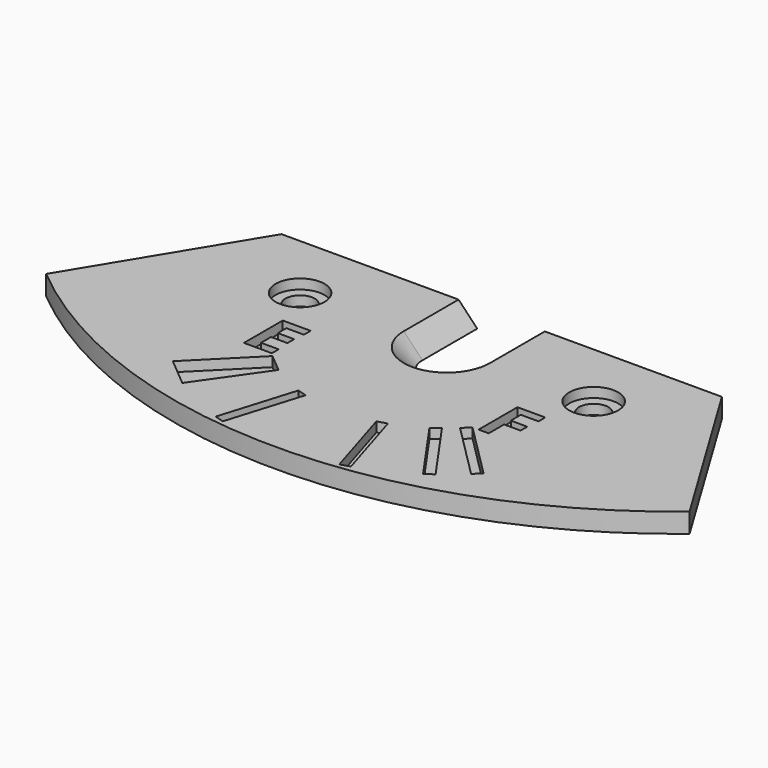
from build123d import *

# Parameters (mm, degrees)
F0_R         = 1.5
F1_DEPTH     = 2
F2_R         = 2.5
F2_R_2       = 1.5
F2_TEXT_SIZE = 6.9444444444
F3_DEPTH     = 1


# Not quite as in the source:
# - Text() gives the source's letters only with a copy of the font that has no kerning and outlines rounded to 1/6400 em; it was checked with that copy


with BuildPart() as f1:
    # F0 (on Top) → F1 (new body)
    with BuildSketch(Plane.XY):
        with BuildLine():
            ThreePointArc((2.5, 0), (0, -2.5), (-2.5, 0))
            Line((-2.5, 0), (-2.5, 7))
            Line((-2.5, 7), (-22.5, 7))
            Line((-22.5, 7), (-32.8723314143, -10.1001386261))
            ThreePointArc((-32.8723314143, -10.1001386261), (0, -22), (32.8723314143, -10.1001386261))
            Line((32.8723314143, -10.1001386261), (22.5, 7))
            Line((22.5, 7), (2.5, 7))
            Line((2.5, 7), (2.5, 0))
        make_face()
        with Locations((-15, 0)):
            Circle(F0_R, mode=Mode.SUBTRACT)
        with Locations((15, 0)):
            Circle(F0_R, mode=Mode.SUBTRACT)
    extrude(amount=F1_DEPTH)

    # F2 (on face) → F3 (cut)
    with BuildSketch(Plane.XY.offset(2)):
        Polygon((-8.0300701089, -11.46812862), (-9.8994949366, -9.8994949366), (-15.5563491861, -15.5563491861), (-12.6186815997, -18.0213449744), align=None)
        Polygon((-3.6150514881, -13.5344524358), (-4.5713562441, -13.2420807311), (-6.9103298819, -20.8925187788), (-5.9540251259, -21.1848904835), align=None)
        Polygon((10.2530483272, -9.545941546), (9.8994949366, -9.8994949366), (15.552331015, -15.552331015), (15.9058844056, -15.1987776244), align=None)
        Polygon((15.552331015, -15.552331015), (9.8994949366, -9.8994949366), (9.545941546, -10.2530483272), (15.1987776244, -15.9058844056), align=None)
        Polygon((6.9103298819, -20.8925187788), (4.5713562441, -13.2420807311), (3.6150514881, -13.5344524358), (5.9540251259, -21.1848904835), align=None)
        Polygon((8.4396461311, -11.1813404019), (7.6204940868, -11.7549168382), (12.2058461996, -18.3034783184), (13.0249982439, -17.729901882), align=None)
        with Locations((-15, 0)):
            Circle(F2_R)
        with Locations((-15, 0)):
            Circle(F2_R_2, mode=Mode.SUBTRACT)
        with Locations((15, 0)):
            Circle(F2_R)
        with Locations((-13.7252705494, -9.545941546)):
            Text('E', F2_TEXT_SIZE, font='Open Sans', font_style=FontStyle.BOLD, text_align=(TextAlign.LEFT, TextAlign.BOTTOM))
        with Locations((10.2530483272, -9.545941546)):
            Text('F', F2_TEXT_SIZE, font='Open Sans', font_style=FontStyle.BOLD, text_align=(TextAlign.LEFT, TextAlign.BOTTOM))
    extrude(amount=-F3_DEPTH, mode=Mode.SUBTRACT)

    # F6 (on offset) → F7 section 0
    with BuildSketch(Plane.XY.offset(2.1)):
        with BuildLine():
            Line((-4.5, 7), (-4.5, 0))
            ThreePointArc((-4.5, 0), (0, -4.5), (4.5, 0))
            Line((4.5, 0), (4.5, 7))
            Line((4.5, 7), (-4.5, 7))
        make_face()
    # F4 (on face) → F7 section 1
    with BuildSketch(Plane.XY):
        with BuildLine():
            Line((2.5, 7), (-2.5, 7))
            Line((-2.5, 7), (-2.5, 0))
            ThreePointArc((-2.5, 0), (0, -2.5), (2.5, 0))
            Line((2.5, 0), (2.5, 7))
        make_face()
    loft(mode=Mode.SUBTRACT)


solid = f1.part
